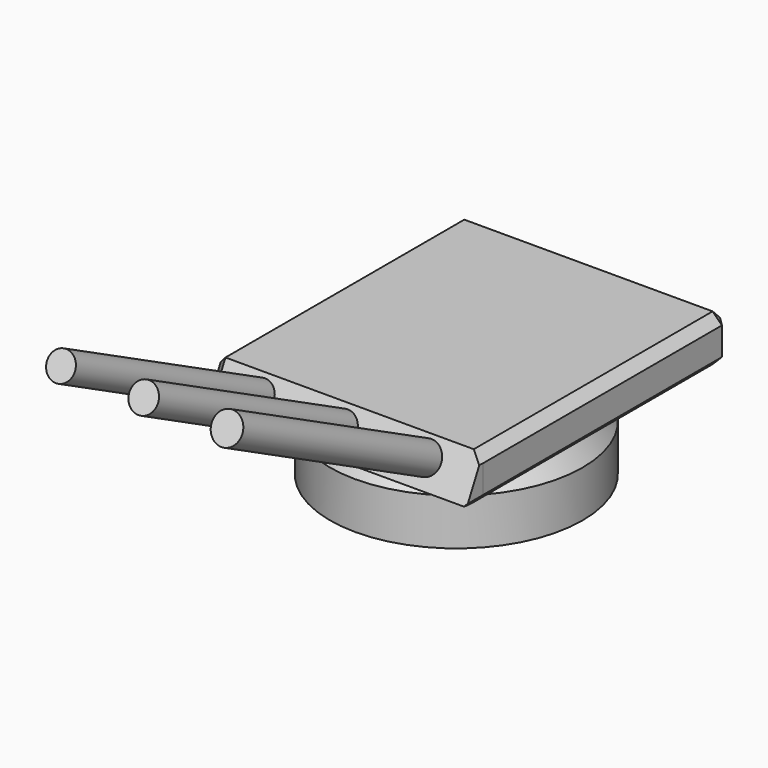
from build123d import *

# Parameters (mm, degrees)
F0_R          = 68.9605399234
F1_DEPTH      = 25.4
F1_FACE_R     = 68.9605399234
F3_R          = 60.7226092801
F6_W          = 145.7738131285
F6_H          = 168.1185737252
F7_DEPTH      = 25.4
F9_DEPTH      = 145.7452
F10_R         = 7.661788512
F11_DEPTH     = 152.4
F10_R_2       = 7.8545121503
F12_DEPTH     = 152.4
F10_R_3       = 8.3767074996
F13_DEPTH     = 152.4
F14_T1_DEPTH  = 6.4524666085
F14_T3_DEPTH  = 6.4524666085
F14_T5_DEPTH  = 6.4524666085
F14_T7_DEPTH  = 6.4524666085
F14_T9_DEPTH  = 194.246872883
F14_T11_DEPTH = 171.9021122862
F14_T13_DEPTH = 51.5282991577
F14_T15_DEPTH = 50.7179530303
F14_T17_DEPTH = 52.9613742976
F14_T19_DEPTH = 203.3917775882


# Not quite as in the source:
# - a fillet or chamfer that OpenCascade refuses, or shapes differently, is made with other operations: its cross-section is extruded or revolved along the edge and cut away or added


with BuildPart() as f1:
    # F0 (on Top) → F1 (new body)
    with BuildSketch(Plane.XY):
        Circle(F0_R)
    extrude(amount=F1_DEPTH)

    # F1_face (on face) → F4 section 0
    with BuildSketch(Plane.XY.offset(25.4)):
        Circle(F1_FACE_R)
    # F3 (on offset) → F4 section 1
    with BuildSketch(Plane.XY.offset(38.1)):
        Circle(F3_R)
    loft()

    # F6 (on offset) → F7 (join)
    with BuildSketch(Plane.XY.offset(38.1)):
        with Locations((0.0197812915, 11.1924894154)):
            Rectangle(F6_W, F6_H)
    extrude(amount=F7_DEPTH)

    # F8 (on face) → F9 (join)
    with BuildSketch(Plane(origin=(-72.8671252728, 0, 0), x_dir=(0, -1, 0), z_dir=(-1, 0, 0))):
        Polygon((84.0455666184, 41.5982604027), (72.8667974472, 63.5), (72.8667974472, 38.1), (81.1657728121, 40.1283976971), align=None)
    extrude(amount=-F9_DEPTH)

    # F10 (on face) → F11 (join)
    with BuildSketch(Plane(origin=(0, -83.5195521199, 42.6288418911), x_dir=(1, 0, 0), z_dir=(0, -0.8906892188, 0.4546127094))):
        with Locations((-45.3161597252, 13.2729420438)):
            Circle(F10_R)
    extrude(amount=F11_DEPTH)

    # F10 (on face) → F12 (join)
    with BuildSketch(Plane(origin=(0, -83.5195521199, 42.6288418911), x_dir=(1, 0, 0), z_dir=(0, -0.8906892188, 0.4546127094))):
        with Locations((0, 12.888232246)):
            Circle(F10_R_2)
    extrude(amount=F12_DEPTH)

    # F10 (on face) → F13 (join)
    with BuildSketch(Plane(origin=(0, -83.5195521199, 42.6288418911), x_dir=(1, 0, 0), z_dir=(0, -0.8906892188, 0.4546127094))):
        with Locations((45.4874783754, 12.888232246)):
            Circle(F10_R_3)
    extrude(amount=F13_DEPTH)

    # F14: chamfer of 5.08 on 11 edges, made by hand

    # F14_s2 → F14_t1 (cut)
    with BuildSketch(Plane(origin=(39.9661547112, 39.9661547112, -39.9661547112), x_dir=(-0.7071067812, 0.7071067812, 0), z_dir=(0.5773502692, 0.5773502692, -0.5773502692))):
        Polygon((19.392465998, 101.8328265585), (15.8003635496, 95.6111226119), (12.2082611012, 101.8328265585), align=None)
    extrude(amount=F14_T1_DEPTH, mode=Mode.SUBTRACT)

    # F14_s4 → F14_t3 (cut)
    with BuildSketch(Plane(origin=(-39.9529671836, 39.9529671836, -39.9529671836), x_dir=(-0.7071067812, -0.7071067812, 0), z_dir=(-0.5773502692, 0.5773502692, -0.5773502692))):
        Polygon((-12.2362360719, 101.8166752017), (-19.4204409687, 101.8166752017), (-15.8283385203, 95.594971255), align=None)
    extrude(amount=F14_T3_DEPTH, mode=Mode.SUBTRACT)

    # F14_s6 → F14_t5 (cut)
    with BuildSketch(Plane(origin=(-73.8196338503, 73.8196338503, 73.8196338503), x_dir=(-0.7071067812, -0.7071067812, 0), z_dir=(-0.5773502692, 0.5773502692, 0.5773502692))):
        Polygon((-12.2362360719, -18.8606225794), (-19.4204409687, -18.8606225794), (-15.8283385203, -12.6389186327), align=None)
    extrude(amount=F14_T5_DEPTH, mode=Mode.SUBTRACT)

    # F14_s8 → F14_t7 (cut)
    with BuildSketch(Plane(origin=(73.8328213779, 73.8328213779, 73.8328213779), x_dir=(-0.7071067812, 0.7071067812, 0), z_dir=(0.5773502692, 0.5773502692, 0.5773502692))):
        Polygon((19.392465998, -18.8767739363), (15.8003635496, -12.6550699896), (12.2082611012, -18.8767739363), align=None)
    extrude(amount=F14_T7_DEPTH, mode=Mode.SUBTRACT)

    # F14_s10 → F14_t9 (cut)
    with BuildSketch(Plane.XZ.offset(-108.3159258569)):
        Polygon((67.8266878557, 38.1), (72.9066878557, 43.18), (72.9066878557, 38.1), align=None)
        Polygon((-72.8671252728, 58.42), (-67.7871252728, 63.5), (-72.8671252728, 63.5), align=None)
        Polygon((67.8266878557, 63.5), (72.9066878557, 58.42), (72.9066878557, 63.5), align=None)
    extrude(amount=F14_T9_DEPTH, mode=Mode.SUBTRACT)

    # F14_s12 → F14_t11 (cut)
    with BuildSketch(Plane.YZ.offset(-85.9312748516)):
        Polygon((95.251776278, 43.18), (90.171776278, 38.1), (95.251776278, 38.1), align=None)
        Polygon((95.251776278, 58.42), (90.171776278, 63.5), (95.251776278, 63.5), align=None)
    extrude(amount=F14_T11_DEPTH, mode=Mode.SUBTRACT)

    # F14_s14 → F14_t13 (cut)
    with BuildSketch(Plane.XY.offset(25.0358504211)):
        Polygon((-72.8671252728, 90.171776278), (-67.7871252728, 95.251776278), (-72.8671252728, 95.251776278), align=None)
        Polygon((67.8266878557, 95.251776278), (72.9066878557, 90.171776278), (72.9066878557, 95.251776278), align=None)
    extrude(amount=F14_T13_DEPTH, mode=Mode.SUBTRACT)

    # F14_s16 → F14_t15 (cut)
    with BuildSketch(Plane(origin=(0, -6.4651429351, -12.6666786706), x_dir=(1, 0, 0), z_dir=(0, 0.4546127094, 0.8906892188))):
        Polygon((-72.8671252728, -88.6895779413), (-67.7871252728, -93.7695779413), (-72.8671252728, -93.7695779413), align=None)
    extrude(amount=F14_T15_DEPTH, mode=Mode.SUBTRACT)

    # F14_s18 → F14_t17 (cut)
    with BuildSketch(Plane(origin=(0, -55.9724859152, 13.6805396495), x_dir=(1, 0, 0), z_dir=(0, -0.9714055055, 0.2374265019))):
        Polygon((-72.8671252728, 24.7900409374), (-67.7871252728, 19.7100409374), (-72.8671252728, 19.7100409374), align=None)
    extrude(amount=F14_T17_DEPTH, mode=Mode.SUBTRACT)

    # F14_s20 → F14_t19 (cut)
    with BuildSketch(Plane.XZ.offset(-108.3159258569)):
        Polygon((-72.8671252728, 43.18), (-67.7871252728, 38.1), (-72.8671252728, 38.1), align=None)
    extrude(amount=F14_T19_DEPTH, mode=Mode.SUBTRACT)


solid = f1.part
